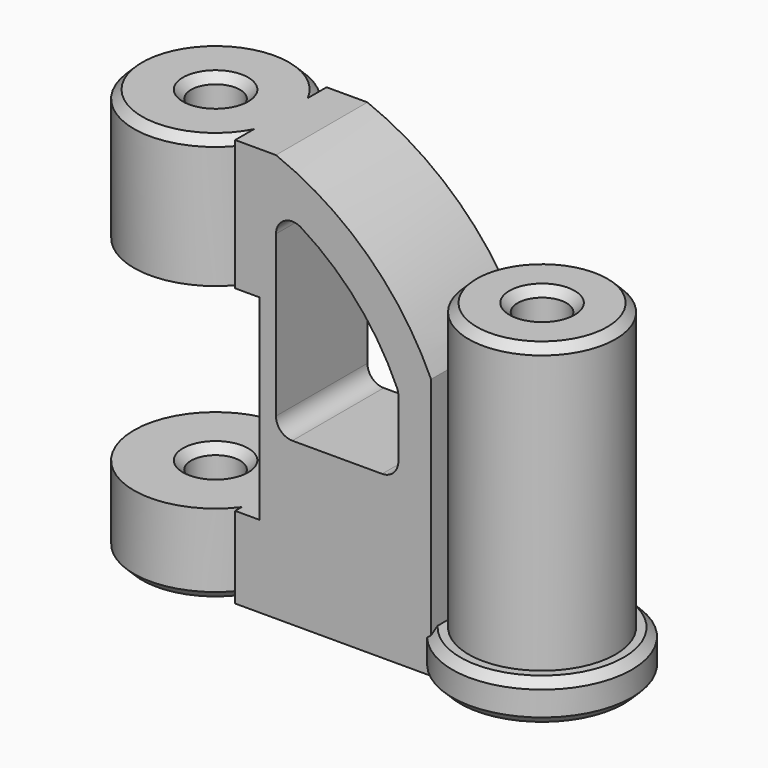
from build123d import *

# Parameters (mm, degrees)
F0_R          = 25.4
F0_R_2        = 7.62
F1_DEPTH      = 127
F0_R_3        = 22.86
F2_DEPTH      = 101.6
F4_DEPTH      = 17.78
F4_DEPTH_BACK = 17.78
F5_W          = 60.96
F5_H          = 60.96
F6_DEPTH      = 25.4
F6_DEPTH_BACK = 25.4
F7_R          = 5.08
F8_T4_ANGLE   = 315.8495903275
F8_T13_ANGLE  = 315.8495903275
F9_R          = 27.94
F9_R_2        = 22.86
F10_DEPTH     = 12.7
F11_SIZE      = 2.54


# Not quite as in the source:
# - a fillet or chamfer that OpenCascade refuses, or shapes differently, is made with other operations: its cross-section is extruded or revolved along the edge and cut away or added


with BuildPart() as f1:
    # F0 (on Top) → F1 (new body)
    with BuildSketch(Plane.XY):
        Circle(F0_R)
        Circle(F0_R_2, mode=Mode.SUBTRACT)
    extrude(amount=F1_DEPTH)



with BuildPart() as f2:
    # F0 (on Top) → F2 (new body)
    with BuildSketch(Plane.XY):
        with Locations((101.6, 0)):
            Circle(F0_R_3)
        with Locations((101.6, 0)):
            Circle(F0_R_2, mode=Mode.SUBTRACT)
    extrude(amount=F2_DEPTH)


with BuildPart() as f1_1:
    add(f1.part)

    add(f2.part)  # F4 merges F2
    # F3 (on Front) → F4 (join, two sides)
    with BuildSketch(Plane.XZ) as f4_sk:
        with BuildLine():
            Line((20.32, 127), (20.32, 0))
            Line((20.32, 0), (81.28, 0))
            Line((81.28, 0), (81.28, 81.28))
            ThreePointArc((81.28, 81.28), (61.5844056789, 108.82076155), (33.02, 127))
            Line((33.02, 127), (20.32, 127))
        make_face()
        with BuildLine():
            Line((33.02, 50.4039023765), (33.02, 113.9039023765))
            ThreePointArc((33.02, 113.9039023765), (55.7015227305, 97.7137904926), (71.12, 74.5008252602))
            Line((71.12, 74.5008252602), (71.12, 50.4039023765))
            Line((71.12, 50.4039023765), (33.02, 50.4039023765))
        make_face(mode=Mode.SUBTRACT)
    extrude(amount=F4_DEPTH)
    extrude(f4_sk.sketch, amount=-F4_DEPTH_BACK)

    # F5 (on Front) → F6 (cut, two sides)
    with BuildSketch(Plane.XZ) as f6_sk:
        with Locations((-2.54, 55.88)):
            Rectangle(F5_W, F5_H)
    extrude(amount=F6_DEPTH, mode=Mode.SUBTRACT)
    extrude(f6_sk.sketch, amount=-F6_DEPTH_BACK, mode=Mode.SUBTRACT)

    # F7
    f7_edges = [f1_1.edges().sort_by_distance(p)[0] for p in [
        (33.02, 0, 113.903902),
        (33.02, 0, 50.403902),
        (71.12, 0, 50.403902),
        (71.12, 0, 74.500825),
    ]]
    fillet(f7_edges, radius=F7_R)

    # F8: chamfer of 2.54 on 4 edges, made by hand


with BuildPart() as f8_tool2:
    # F8_s3 → F8_t4 (revolve)
    with BuildSketch(Plane(origin=(0, 0, 0), x_dir=(0, 0, 1), z_dir=(0.3758232659, -0.9266913579, 0))):
        Polygon((0, -22.86), (2.54, -25.4), (0, -25.4), align=None)
    revolve(axis=Axis((0, 0, 0), (0, 0, 1)), revolution_arc=F8_T4_ANGLE)

    split(bisect_by=Plane.YZ.offset(20.32), keep=Keep.BOTTOM)


with BuildPart() as f1_2:
    add(f1_1.part)

    # F8_t1: cut F8_tool2
    add(f8_tool2.part, mode=Mode.SUBTRACT)

    # F8_s6 → F8_t7 (revolve, cut)
    with BuildSketch(Plane.XZ):
        Polygon((10.16, 25.4), (7.62, 22.86), (7.62, 25.4), align=None)
    revolve(axis=Axis((0, 0, 25.4), (0, 0, -1)), mode=Mode.SUBTRACT)

    # F8_s8 → F8_t9 (revolve, cut)
    with BuildSketch(Plane.XZ):
        Polygon((10.16, 86.36), (7.62, 88.9), (7.62, 86.36), align=None)
    revolve(axis=Axis((0, 0, 86.36), (0, 0, -1)), mode=Mode.SUBTRACT)


with BuildPart() as f8_tool11:
    # F8_s12 → F8_t13 (revolve)
    with BuildSketch(Plane(origin=(0, 0, 0), x_dir=(0, 0, 1), z_dir=(0.3758232659, -0.9266913579, 0))):
        Polygon((127, -22.86), (124.46, -25.4), (127, -25.4), align=None)
    revolve(axis=Axis((0, 0, 127), (0, 0, 1)), revolution_arc=F8_T13_ANGLE)

    split(bisect_by=Plane.YZ.offset(20.32), keep=Keep.BOTTOM)


with BuildPart() as f1_3:
    add(f1_2.part)

    # F8_t10: cut F8_tool11
    add(f8_tool11.part, mode=Mode.SUBTRACT)

    # F9 (on Top) → F10 (join)
    with BuildSketch(Plane.XY):
        with Locations((101.6, 0)):
            Circle(F9_R)
        with Locations((101.6, 0)):
            Circle(F9_R_2, mode=Mode.SUBTRACT)
    extrude(amount=F10_DEPTH)

    # F11
    f11_edges = [f1_3.edges().sort_by_distance(p)[0] for p in [
        (129.54, 0, 0),
        (129.54, 0, 12.7),
        (78.74, 0, 101.6),
        (93.98, 0, 101.6),
        (-7.62, 0, 127),
    ]]
    chamfer(f11_edges, length=F11_SIZE)


solid = f1_3.part
